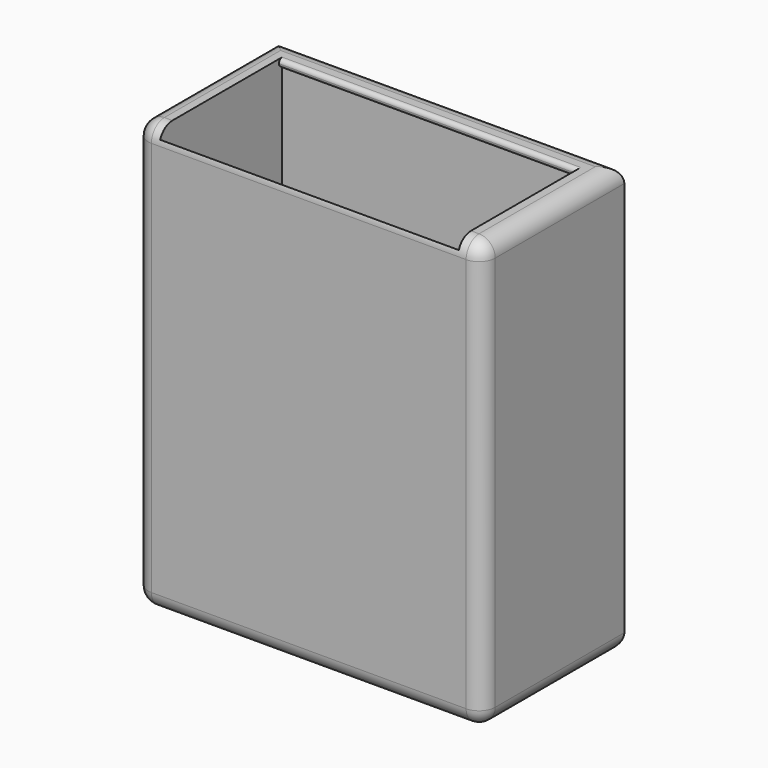
from build123d import *

# Parameters (mm, degrees)
F0_W        = 43
F0_H        = 22
F1_DEPTH    = 53
F2_T        = -3
F3_W        = 37
F3_H        = 0.5
F4_DEPTH    = 1
F5_R        = 0.49999
F6_R        = 2
F7_T1_DEPTH = 37


# Not quite as in the source:
# - a fillet or chamfer that OpenCascade refuses, or shapes differently, is made with other operations: its cross-section is extruded or revolved along the edge and cut away or added
# - a fillet or chamfer is up to 0.001 mm smaller than in the source, because OpenCascade refuses the exact size


with BuildPart() as f1:
    # F0 (on Top) → F1 (new body)
    with BuildSketch(Plane.XY):
        Rectangle(F0_W, F0_H)
    extrude(amount=F1_DEPTH)

    # F2
    f2_openings = [f1.faces().sort_by_distance(p)[0] for p in [
        (0, 0, 53),
    ]]
    offset(amount=F2_T, openings=f2_openings)

    # F3 (on face) → F4 (join)
    with BuildSketch(Plane.XY.offset(53)):
        with Locations((0, 7.75)):
            Rectangle(F3_W, F3_H)
    extrude(amount=-F4_DEPTH)

    # F5 (radius 0.5 in the source; OpenCascade refuses exactly that, so slightly less here)
    f5_edges = [f1.edges().sort_by_distance(p)[0] for p in [
        (0, 7.5, 53),
        (0, 7.5, 52),
    ]]
    fillet(f5_edges, radius=F5_R)

    # F6
    f6_edges = [f1.edges().sort_by_distance(p)[0] for p in [
        (21.5, -11, 26.5),
        (-21.5, -11, 26.5),
        (21.5, 0, 0),
        (0, 11, 0),
        (-21.5, 0, 0),
        (0, -11, 0),
        (-21.5, 0, 53),
        (0, 11, 53),
        (21.5, 0, 53),
        (0, -11, 53),
    ]]
    fillet(f6_edges, radius=F6_R)

    # F7: fillet of radius 7 on 1 edges, made by hand

    # F7_s2 → F7_t1 (cut)
    with BuildSketch(Plane.YZ.offset(-18.5)):
        with BuildLine():
            ThreePointArc((-15, 53), (-10.0502525317, 50.9497474683), (-8, 46))
            Line((-8, 46), (-7.86, 46))
            Line((-7.86, 46), (-7.86, 53.14))
            Line((-7.86, 53.14), (-15, 53.14))
            Line((-15, 53.14), (-15, 53))
        make_face()
    extrude(amount=F7_T1_DEPTH, mode=Mode.SUBTRACT)


solid = f1.part
